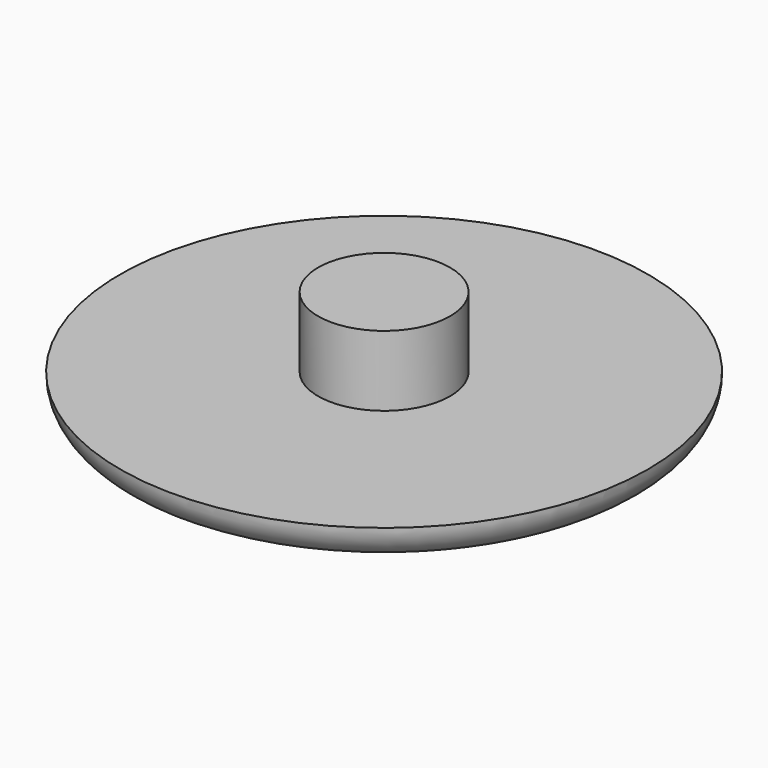
from build123d import *

# Parameters (mm, degrees)
F0_R     = 15
F0_R_2   = 3.75
F1_DEPTH = 2
F2_R     = 3.75
F3_DEPTH = 4
F4_R     = 1.99999


# Not quite as in the source:
# - a fillet or chamfer is up to 0.001 mm smaller than in the source, because OpenCascade refuses the exact size


with BuildPart() as f1:
    # F0 (on Top) → F1 (new body)
    with BuildSketch(Plane.XY):
        Circle(F0_R)
        Circle(F0_R_2, mode=Mode.SUBTRACT)
        Circle(F0_R_2)
    extrude(amount=F1_DEPTH)

    # F2 (on face) → F3 (join)
    with BuildSketch(Plane.XY.offset(2)):
        Circle(F2_R)
    extrude(amount=F3_DEPTH)

    # F4 (radius 2 in the source; OpenCascade refuses exactly that, so slightly less here)
    f4_edges = [f1.edges().sort_by_distance(p)[0] for p in [
        (-15, 0, 0),
    ]]
    fillet(f4_edges, radius=F4_R)


solid = f1.part
